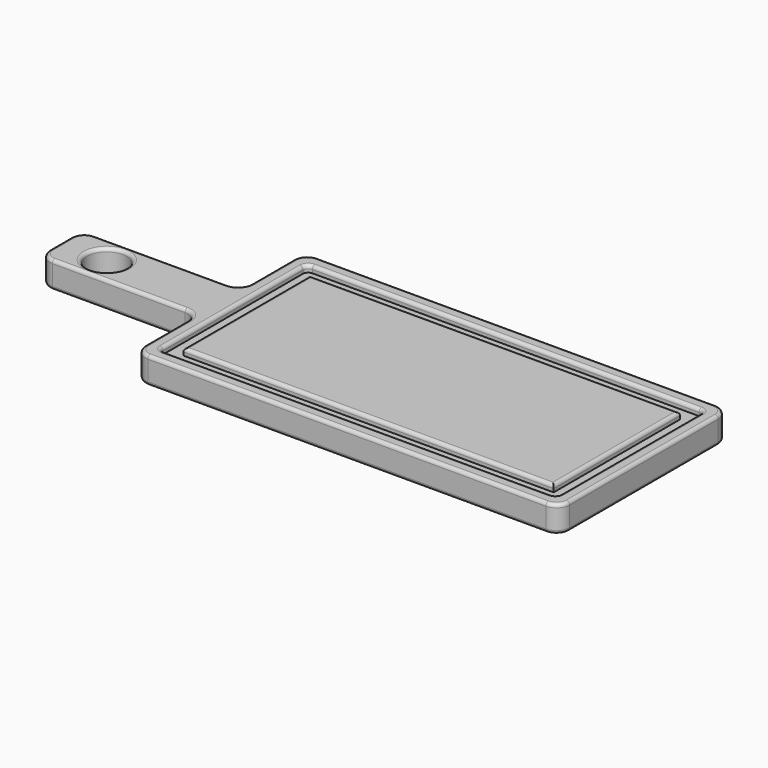
from build123d import *

# Parameters (mm, degrees)
F0_W     = 152.4
F0_H     = 50.8
F1_DEPTH = 25.4
F2_R     = 19.05
F3_DEPTH = 25.4
F5_DEPTH = 6.35
F6_R     = 12.7
F7_R     = 5.08
F8_R     = 3.17499


# Not quite as in the source:
# - a fillet or chamfer is up to 0.001 mm smaller than in the source, because OpenCascade refuses the exact size


with BuildPart() as f1:
    # F0 (on Top) → F1 (new body)
    with BuildSketch(Plane.XY):
        Polygon((0, 76.2), (0, 0), (406.4, 0), (406.4, 203.2), (0, 203.2), (0, 127), align=None)
        with Locations((-76.2, 101.6)):
            Rectangle(F0_W, F0_H)
    extrude(amount=F1_DEPTH)

    # F2 (on face) → F3 (cut)
    with BuildSketch(Plane.XY.offset(25.4)):
        with Locations((-107.95, 101.6)):
            Circle(F2_R)
    extrude(amount=-F3_DEPTH, mode=Mode.SUBTRACT)

    # F4 (on face) → F5 (cut)
    with BuildSketch(Plane.XY.offset(25.4)):
        Polygon((12.953999114, 76.2), (12.953999114, 12.953999114), (393.446000886, 12.953999114), (393.446000886, 190.246000886), (12.953999114, 190.246000886), (12.953999114, 127), align=None)
        Polygon((25.9079957724, 76.2), (25.9079957724, 127), (25.9079957724, 177.2920042276), (380.4920042276, 177.2920042276), (380.4920042276, 25.9079957724), (25.9079957724, 25.9079957724), align=None, mode=Mode.SUBTRACT)
    extrude(amount=-F5_DEPTH, mode=Mode.SUBTRACT)

    # F6
    f6_edges = [f1.edges().sort_by_distance(p)[0] for p in [
        (-152.4, 76.2, 12.7),
        (-152.4, 127, 12.7),
        (0, 203.2, 12.7),
        (0, 0, 12.7),
        (406.4, 203.2, 12.7),
        (406.4, 0, 12.7),
        (0, 76.2, 12.7),
        (0, 127, 12.7),
    ]]
    fillet(f6_edges, radius=F6_R)

    # F7
    f7_edges = [f1.edges().sort_by_distance(p)[0] for p in [
        (12.953999, 190.246001, 22.225),
        (393.446001, 190.246001, 22.225),
        (393.446001, 12.953999, 22.225),
        (12.953999, 12.953999, 22.225),
    ]]
    fillet(f7_edges, radius=F7_R)

    # F8 (radius 3.175 in the source; OpenCascade refuses exactly that, so slightly less here)
    f8_edges = [f1.edges().sort_by_distance(p)[0] for p in [
        (203.2, 177.292004, 25.4),
        (380.492004, 101.6, 25.4),
        (203.2, 25.907996, 25.4),
        (25.907996, 101.6, 25.4),
        (203.2, 12.953999, 25.4),
        (14.441897, 14.441897, 25.4),
        (391.958103, 14.441897, 25.4),
        (12.953999, 101.6, 25.4),
        (393.446001, 101.6, 25.4),
        (14.441897, 188.758103, 25.4),
        (391.958103, 188.758103, 25.4),
        (203.2, 190.246001, 25.4),
        (0, 38.1, 25.4),
        (-3.719744, 72.480256, 25.4),
        (3.719744, 3.719744, 25.4),
        (-76.2, 76.2, 25.4),
        (203.2, 0, 25.4),
        (-148.680256, 79.919744, 25.4),
        (402.680256, 3.719744, 25.4),
        (-152.4, 101.6, 25.4),
        (406.4, 101.6, 25.4),
        (-148.680256, 123.280256, 25.4),
        (402.680256, 199.480256, 25.4),
        (-76.2, 127, 25.4),
        (203.2, 203.2, 25.4),
        (-3.719744, 130.719744, 25.4),
        (3.719744, 199.480256, 25.4),
        (0, 165.1, 25.4),
        (-127, 101.6, 25.4),
        (0, 38.1, 0),
        (-3.719744, 72.480256, 0),
        (3.719744, 3.719744, 0),
        (-76.2, 76.2, 0),
        (203.2, 0, 0),
        (-148.680256, 79.919744, 0),
        (402.680256, 3.719744, 0),
        (-152.4, 101.6, 0),
        (406.4, 101.6, 0),
        (-148.680256, 123.280256, 0),
        (402.680256, 199.480256, 0),
        (-76.2, 127, 0),
        (203.2, 203.2, 0),
        (-3.719744, 130.719744, 0),
        (3.719744, 199.480256, 0),
        (0, 165.1, 0),
        (-127, 101.6, 0),
    ]]
    fillet(f8_edges, radius=F8_R)


solid = f1.part
